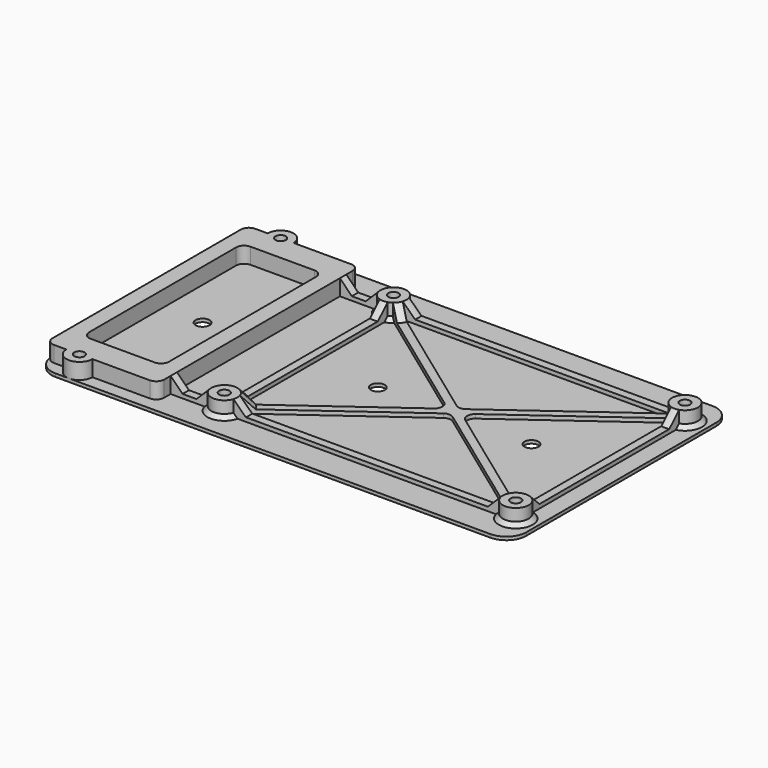
from build123d import *

# Parameters (mm, degrees)
F3_DEPTH  = 4
F5_DEPTH  = 1
F6_R      = 3.25
F7_DEPTH  = 4
F8_W      = 118.9
F8_H      = 69.5
F9_DEPTH  = 0.8
F10_R     = 5
F11_D     = 2.6
F11_DEPTH = 4.001
F12_SIZE  = 2.99999
F13_SIZE  = 1
F14_D     = 3.5


# Not quite as in the source:
# - a fillet or chamfer is up to 0.001 mm smaller than in the source, because OpenCascade refuses the exact size
# - after a boolean that leaves OpenCascade's solid faulty, fix() repairs it


with BuildPart() as f3:
    # F2 (on Top) → F3 (new body)
    with BuildSketch(Plane.XY):
        with BuildLine():
            Line((12, 31.5), (-12, 31.5))
            ThreePointArc((-12, 31.5), (-13.4142135624, 30.9142135624), (-14, 29.5))
            Line((-14, 29.5), (-14, -29.5))
            ThreePointArc((-14, -29.5), (-13.4142135624, -30.9142135624), (-12, -31.5))
            Line((-12, -31.5), (12, -31.5))
            ThreePointArc((12, -31.5), (13.4142135624, -30.9142135624), (14, -29.5))
            Line((14, -29.5), (14, 29.5))
            ThreePointArc((14, 29.5), (13.4142135624, 30.9142135624), (12, 31.5))
        make_face()
        with BuildLine():
            ThreePointArc((10, -23), (9.4142135624, -24.4142135624), (8, -25))
            Line((8, -25), (-8, -25))
            ThreePointArc((-8, -25), (-9.4142135624, -24.4142135624), (-10, -23))
            Line((-10, -23), (-10, 23))
            ThreePointArc((-10, 23), (-9.4142135624, 24.4142135624), (-8, 25))
            Line((-8, 25), (8, 25))
            ThreePointArc((8, 25), (9.4142135624, 24.4142135624), (10, 23))
            Line((10, 23), (10, -23))
        make_face(mode=Mode.SUBTRACT)
    extrude(amount=F3_DEPTH)

    # F4 (on Top) → F5 (join)
    with BuildSketch(Plane.XY):
        with BuildLine():
            ThreePointArc((100.65, 26.5), (100.3571067812, 27.2071067812), (99.65, 27.5))
            Line((99.65, 27.5), (14, 27.5))
            ThreePointArc((14, 27.5), (13, 26.5), (14, 25.5))
            Line((14, 25.5), (25.65, 25.5))
            Line((25.65, 25.5), (25.65, -25.5))
            Line((25.65, -25.5), (14, -25.5))
            ThreePointArc((14, -25.5), (13, -26.5), (14, -27.5))
            Line((14, -27.5), (99.65, -27.5))
            ThreePointArc((99.65, -27.5), (100.3571067812, -27.2071067812), (100.65, -26.5))
            Line((100.65, -26.5), (100.65, 26.5))
        make_face()
        with BuildLine():
            Line((64.3250247719, -2.0888654384), (96.5705497341, -25.5))
            Line((96.5705497341, -25.5), (29.7294502659, -25.5))
            Line((29.7294502659, -25.5), (61.9749752281, -2.0888654384))
            ThreePointArc((61.9749752281, -2.0888654384), (63.15, -1.7072957846), (64.3250247719, -2.0888654384))
        make_face(mode=Mode.SUBTRACT)
        with BuildLine():
            Line((59.218749446, -1.6184303462), (27.65, -24.5382073412))
            Line((27.65, -24.5382073412), (27.65, 24.5382073412))
            Line((27.65, 24.5382073412), (59.218749446, 1.6184303462))
            ThreePointArc((59.218749446, 1.6184303462), (60.0437246741, 0), (59.218749446, -1.6184303462))
        make_face(mode=Mode.SUBTRACT)
        with BuildLine():
            Line((61.9749752281, 2.0888654384), (29.7294502659, 25.5))
            Line((29.7294502659, 25.5), (96.5705497341, 25.5))
            Line((96.5705497341, 25.5), (64.3250247719, 2.0888654384))
            ThreePointArc((64.3250247719, 2.0888654384), (63.15, 1.7072957846), (61.9749752281, 2.0888654384))
        make_face(mode=Mode.SUBTRACT)
        with BuildLine():
            Line((67.081250554, 1.6184303462), (98.65, 24.5382073412))
            Line((98.65, 24.5382073412), (98.65, -24.5382073412))
            Line((98.65, -24.5382073412), (67.081250554, -1.6184303462))
            ThreePointArc((67.081250554, -1.6184303462), (66.2562753259, 0), (67.081250554, 1.6184303462))
        make_face(mode=Mode.SUBTRACT)
    extrude(amount=F5_DEPTH)

    # F6 (on face) → F7 (join)
    with BuildSketch(Plane(origin=(0, 0, 0), x_dir=(1, 0, 0), z_dir=(0, 0, -1))):
        with Locations((-5.65, -31.5)):
            Circle(F6_R)
        with Locations((-5.65, 31.5)):
            Circle(F6_R)
        with Locations((99.65, 26.5)):
            Circle(F6_R)
        with Locations((99.65, -26.5)):
            Circle(F6_R)
        with Locations((26.65, -26.5)):
            Circle(F6_R)
        with Locations((26.65, 26.5)):
            Circle(F6_R)
    extrude(amount=-F7_DEPTH)

    # F8 (on Top) → F9 (join)
    with BuildSketch(Plane.XY):
        with Locations((45.45, 0)):
            Rectangle(F8_W, F8_H)
    extrude(amount=-F9_DEPTH)

    # F10
    f10_edges = [f3.edges().sort_by_distance(p)[0] for p in [
        (-14, -34.75, -0.4),
        (-14, 34.75, -0.4),
        (104.9, 34.75, -0.4),
        (104.9, -34.75, -0.4),
    ]]
    fillet(f10_edges, radius=F10_R)

    # F11 (through all, one way)
    with BuildSketch(Plane(origin=(0, 0, 0), x_dir=(1, 0, 0), z_dir=(0, 0, -1))):
        with Locations((99.65, -26.5), (26.65, -26.5), (-5.65, -31.5), (-5.65, 31.5), (26.65, 26.5), (99.65, 26.5)):
            Circle(F11_D / 2)
    extrude(amount=-F11_DEPTH, mode=Mode.SUBTRACT)

    # F12 (size 3 in the source; OpenCascade refuses exactly that, so slightly less here)
    f12_edges = [f3.edges().sort_by_distance(p)[0] for p in [
        (29.279949, -24.590585, 1),
        (29.279949, 24.590585, 1),
        (97.020051, -24.590585, 1),
        (14, -26.5, 1),
        (14, 26.5, 1),
        (29.86034, -27.006177, 1),
        (23.4, -26.5, 1),
        (26.65, -23.25, 1),
        (29.86034, -25.993823, 1),
        (96.4, -26.5, 1),
        (99.65, -23.25, 1),
        (29.86034, 25.993823, 1),
        (26.65, 23.25, 1),
        (23.4, 26.5, 1),
        (29.86034, 27.006177, 1),
        (99.65, 23.25, 1),
    ]]
    chamfer(f12_edges, length=F12_SIZE)

    # F13
    f13_edges = [f3.edges().sort_by_distance(p)[0] for p in [
        (24.351903, 24.201903, 0),
        (28.125957, 23.604478, 0),
        (26.65, 29.75, 0),
        (26.65, -29.75, 0),
        (24.351903, -24.201903, 0),
        (28.125957, -23.604478, 0),
        (102.277975, -24.587868, 0),
        (98.174043, -23.604478, 0),
        (100.156177, 29.71034, 0),
        (98.174043, 23.604478, 0),
        (100.156177, -29.71034, 0),
        (102.277975, 24.587868, 0),
    ]]
    chamfer(f13_edges, length=F13_SIZE)

    # F14 (through all)
    with Locations(Plane.XY):
        with Locations((0, 0), (43.9, 0), (82.4, 0)):
            Hole(F14_D / 2)

    add(f3.part.fix(), mode=Mode.REPLACE)


solid = f3.part
